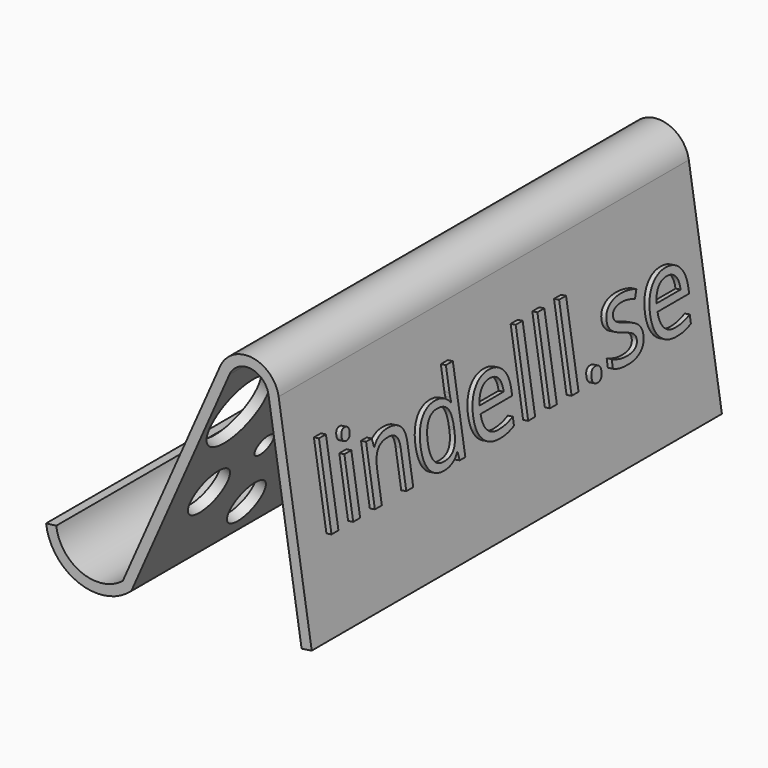
from build123d import *

# Parameters (mm, degrees)
F1_DEPTH     = 50
F2_TEXT_SIZE = 20.9089589081
F3_DEPTH     = 1
F4_R         = 7.0759697278
F4_R_2       = 4.5024899467
F4_R_3       = 4.8677032012
F4_R_4       = 4.0449973846
F4_R_5       = 4.3957429255
F4_R_6       = 7.4894108319
F4_R_7       = 4.3452426111
F4_R_8       = 3.7863953719
F4_R_9       = 4.2471978851
F4_R_10      = 2.9260651907
F4_R_11      = 2.1397737727
F4_R_12      = 4.5953503189
F4_R_13      = 6.9857044068
F4_R_14      = 3.3325672414
F5_DEPTH     = 2.5784799127


# Not quite as in the source:
# - Text() gives the source's letters only with a copy of the font that has no kerning and outlines rounded to 1/6400 em; it was checked with that copy


with BuildPart() as f1:
    # F0 (on Front) → F1 (new body, symmetric)
    with BuildSketch(Plane.XZ):
        with BuildLine():
            Line((-8.2692852635, 43.0005926952), (-27.2416079431, 0))
            ThreePointArc((-27.2416079431, 0), (-35.2783464481, -1.2012912484), (-40.2202455889, 5.2492823185))
            Line((-40.2202455889, 5.2492823185), (-42.2056178482, 5.007834618))
            ThreePointArc((-42.2056178482, 5.007834618), (-35.791265337, -3.1477406677), (-25.5954397788, -1.2235609551))
            Line((-25.5954397788, -1.2235609551), (-6.4394728084, 42.1932598152))
            ThreePointArc((-6.4394728084, 42.1932598152), (-2.2589366232, 44.5445304445), (1.1726152172, 41.1934398259))
            Line((1.1726152172, 41.1934398259), (7.6284958093, -0.3074228853))
            Line((7.6284958093, -0.3074228853), (9.6047273669, 0))
            Line((9.6047273669, 0), (3.1488467749, 41.5008627113))
            ThreePointArc((3.1488467749, 41.5008627113), (-1.9984809858, 46.5274986392), (-8.2692852635, 43.0005926952))
        make_face()
    extrude(amount=F1_DEPTH, both=True)

    # F2 (on face) → F3 (join)
    with BuildSketch(Plane(origin=(9.3777944794, 0, 1.4588111529), x_dir=(0, 1, 0), z_dir=(0.9881157788, 0, 0.1537114427))):
        with Locations((-45, 15.2493364666)):
            Text('lindelll.se', F2_TEXT_SIZE, font='Open Sans', text_align=(TextAlign.LEFT, TextAlign.BOTTOM))
    extrude(amount=F3_DEPTH)

    # F4 (on face) → F5 (cut, through all)
    with BuildSketch(Plane(origin=(-22.8026806926, 0, 10.0607872809), x_dir=(0, -1, 0), z_dir=(-0.9149062276, 0, 0.40366644))):
        with Locations((-31.1241000891, 21.6476190835)):
            Circle(F4_R)
        with Locations((-43.4794910252, 29.8793371767)):
            Circle(F4_R_2)
        with BuildLine():
            ThreePointArc((-50, -5.4229172937), (-38.1257365537, -8.7894708007), (-30.9978231044, 1.2864740565))
            ThreePointArc((-30.9978231044, 1.2864740565), (-38.1257365537, 11.3624189137), (-50, 7.9958654067))
            Line((-50, 7.9958654067), (-50, -5.4229172937))
        make_face()
        with Locations((-20.2282033861, 2.4375929497)):
            Circle(F4_R_3)
        with Locations((-6.3134585507, -5.523249507)):
            Circle(F4_R_4)
        with Locations((-10.4970028624, 17.800251022)):
            Circle(F4_R_5)
        with BuildLine():
            ThreePointArc((-15.6118032551, 36.0034771019), (-19.4747950882, 38.0717330913), (-23.3377869213, 36.0034771019))
            Line((-23.3377869213, 36.0034771019), (-15.6118032551, 36.0034771019))
        make_face()
        with Locations((3.8258717395, 23.7063746899)):
            Circle(F4_R_6)
        with Locations((1.2423713924, 8.3221681416)):
            Circle(F4_R_7)
        with Locations((13.7944864109, -0.8908899617)):
            Circle(F4_R_8)
        with Locations((25.352511555, -4.6541793272)):
            Circle(F4_R_9)
        with Locations((16.3642447442, 11.5187074989)):
            Circle(F4_R_10)
        with Locations((27.9674362391, 9.1007659212)):
            Circle(F4_R_11)
        with Locations((39.2174571753, 4.7142952681)):
            Circle(F4_R_12)
        with Locations((41.4857380092, 23.5361084342)):
            Circle(F4_R_13)
        with Locations((27.0234141499, 21.172426641)):
            Circle(F4_R_14)
        with BuildLine():
            Line((24.7438336078, 36.0034771019), (15.2464797434, 36.0034771019))
            ThreePointArc((15.2464797434, 36.0034771019), (17.6257725811, 25.560271565), (26.476251176, 31.592734158))
            ThreePointArc((26.476251176, 31.592734158), (26.0276192686, 33.9621182525), (24.7438336078, 36.0034771019))
        make_face()
        with BuildLine():
            ThreePointArc((24.7438336078, 36.0034771019), (19.9951566756, 38.0738286585), (15.2464797434, 36.0034771019))
            Line((15.2464797434, 36.0034771019), (24.7438336078, 36.0034771019))
        make_face()
        with BuildLine():
            Line((-15.6118032551, 36.0034771019), (-23.3377869213, 36.0034771019))
            ThreePointArc((-23.3377869213, 36.0034771019), (-20.8191262419, 28.9872981364), (-14.8331093301, 33.4300473332))
            ThreePointArc((-14.8331093301, 33.4300473332), (-15.0320458913, 34.7743784869), (-15.6118032551, 36.0034771019))
        make_face()
    extrude(amount=-F5_DEPTH, mode=Mode.SUBTRACT)


solid = f1.part
